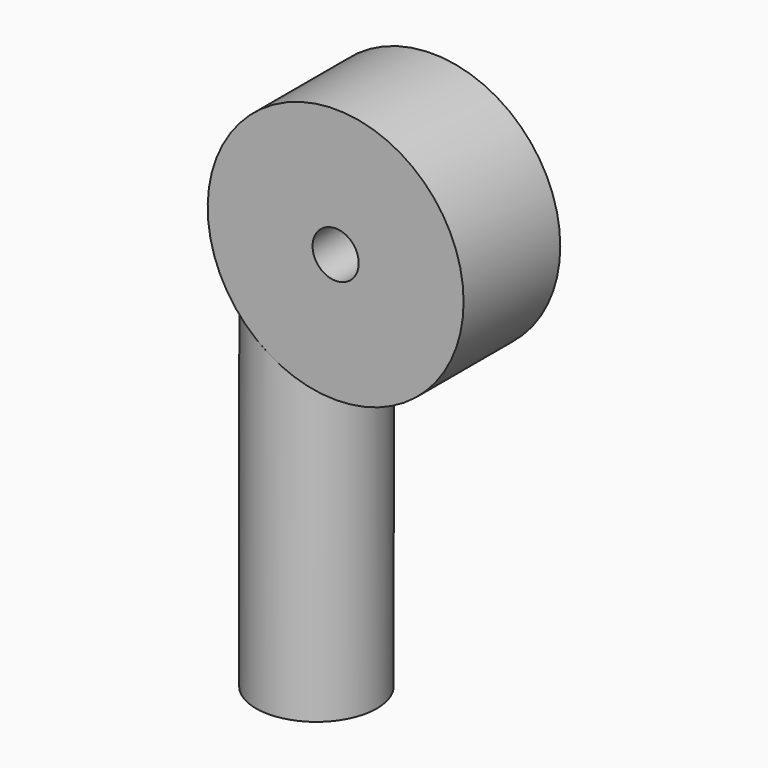
from build123d import *

# Parameters (mm, degrees)
F1_R          = 18
F1_R_2        = 3.25
F2_DEPTH      = 7.5
F2_DEPTH_BACK = 9.5
F3_R          = 8.5
F3_R_2        = 5.225
F4_DEPTH      = 60
F5_DEPTH      = 60.0010001
F5_DEPTH_BACK = 3
F6_DEPTH      = 7.5010001009
F6_DEPTH_BACK = 9.5010001
F8_DEPTH      = 50


# Not quite as in the source:
# - a feature of the source that left no trace in its solid (it failed there, or was rolled back) is left out


with BuildPart() as f2:
    # F1 (on Front) → F2 (new body, two sides)
    with BuildSketch(Plane.XZ) as f2_sk:
        Circle(F1_R)
        Circle(F1_R_2, mode=Mode.SUBTRACT)
    extrude(amount=F2_DEPTH)
    extrude(f2_sk.sketch, amount=-F2_DEPTH_BACK)

    # F3 (on Top) → F4 (join)
    with BuildSketch(Plane.XY):
        with Locations((-9.5, 1)):
            Circle(F3_R)
        with Locations((-9.5, 1)):
            Circle(F3_R_2, mode=Mode.SUBTRACT)
        with Locations((-9.5, 1)):
            Circle(F3_R_2)
    extrude(amount=-F4_DEPTH)

    # F3 (on Top) → F5 (cut, two sides)
    with BuildSketch(Plane.XY) as f5_sk:
        with Locations((-9.5, 1)):
            Circle(F3_R_2)
    extrude(amount=-F5_DEPTH, mode=Mode.SUBTRACT)
    extrude(f5_sk.sketch, amount=F5_DEPTH_BACK, mode=Mode.SUBTRACT)

    # F1 (on Front) → F6 (cut, two sides)
    with BuildSketch(Plane.XZ) as f6_sk:
        Circle(F1_R_2)
    extrude(amount=F6_DEPTH, mode=Mode.SUBTRACT)
    extrude(f6_sk.sketch, amount=-F6_DEPTH_BACK, mode=Mode.SUBTRACT)

    # F1 (on Front) → F8 (cut, symmetric)
    with BuildSketch(Plane.XZ):
        Circle(F1_R_2)
    extrude(amount=F8_DEPTH, both=True, mode=Mode.SUBTRACT)


solid = f2.part
